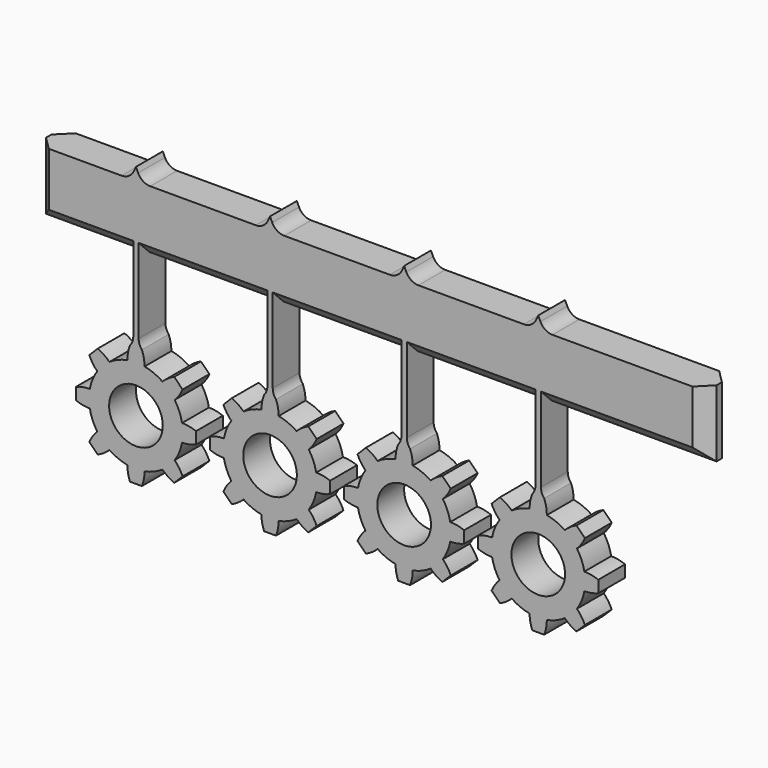
from build123d import *

# Parameters (mm, degrees)
F0_R        = 20
F1_DEPTH    = 12.5
F2_T1_DEPTH = 25
F3_SIZE     = 10


# Not quite as in the source:
# - a fillet or chamfer that OpenCascade refuses, or shapes differently, is made with other operations: its cross-section is extruded or revolved along the edge and cut away or added


with BuildPart() as f1:
    # F0 (on Front) → F1 (new body, symmetric)
    with BuildSketch(Plane.XZ):
        with BuildLine():
            Line((-179.3122274792, 25), (-250, 25))
            Line((-250, 25), (-250, -25))
            Line((-250, -25), (-176.9859883016, -25))
            Line((-176.9859883016, -25), (-176.9859883016, -84.3688530594))
            Line((-176.9859883016, -84.3688530594), (-179.4126922304, -84.3688530594))
            ThreePointArc((-179.4126922304, -84.3688530594), (-180.9081176397, -89.4526936309), (-181.4126922304, -94.727836908))
            ThreePointArc((-181.4126922304, -94.727836908), (-188.3799084344, -96.7969581037), (-194.7695638868, -100.260434299))
            ThreePointArc((-194.7695638868, -100.260434299), (-198.8564415844, -96.8871328307), (-203.5086851747, -94.3497401358))
            Line((-203.5086851747, -94.3497401358), (-209.7689899075, -100.6100448685))
            ThreePointArc((-209.7689899075, -100.6100448685), (-207.2315972126, -105.2622884588), (-203.8582957443, -109.3491661564))
            ThreePointArc((-203.8582957443, -109.3491661564), (-207.3217719395, -115.7388216089), (-209.3908931352, -122.7060378128))
            ThreePointArc((-209.3908931352, -122.7060378128), (-214.6660364123, -123.2106124035), (-219.7498769839, -124.7060378128))
            Line((-219.7498769839, -124.7060378128), (-219.7498769839, -133.5594456704))
            ThreePointArc((-219.7498769839, -133.5594456704), (-214.6660364123, -135.0548710798), (-209.3908931352, -135.5594456704))
            ThreePointArc((-209.3908931352, -135.5594456704), (-207.3217719395, -142.5266618744), (-203.8582957443, -148.9163173268))
            ThreePointArc((-203.8582957443, -148.9163173268), (-207.2315972126, -153.0031950245), (-209.7689899075, -157.6554386148))
            Line((-209.7689899075, -157.6554386148), (-203.5086851747, -163.9157433475))
            ThreePointArc((-203.5086851747, -163.9157433475), (-198.8564415844, -161.3783506526), (-194.7695638868, -158.0050491843))
            ThreePointArc((-194.7695638868, -158.0050491843), (-188.3799084344, -161.4685253795), (-181.4126922304, -163.5376465753))
            ThreePointArc((-181.4126922304, -163.5376465753), (-180.9081176397, -168.8127898524), (-179.4126922304, -173.8966304239))
            Line((-179.4126922304, -173.8966304239), (-170.5592843728, -173.8966304239))
            ThreePointArc((-170.5592843728, -173.8966304239), (-169.0638589634, -168.8127898524), (-168.5592843728, -163.5376465753))
            ThreePointArc((-168.5592843728, -163.5376465753), (-161.5920681688, -161.4685253795), (-155.2024127164, -158.0050491843))
            ThreePointArc((-155.2024127164, -158.0050491843), (-151.1155350188, -161.3783506526), (-146.4632914284, -163.9157433475))
            Line((-146.4632914284, -163.9157433475), (-140.2029866957, -157.6554386148))
            ThreePointArc((-140.2029866957, -157.6554386148), (-142.7403793906, -153.0031950245), (-146.1136808589, -148.9163173268))
            ThreePointArc((-146.1136808589, -148.9163173268), (-142.6502046637, -142.5266618744), (-140.581083468, -135.5594456704))
            ThreePointArc((-140.581083468, -135.5594456704), (-135.3059401909, -135.0548710798), (-130.2220996193, -133.5594456704))
            Line((-130.2220996193, -133.5594456704), (-130.2220996193, -124.7060378128))
            ThreePointArc((-130.2220996193, -124.7060378128), (-135.3059401909, -123.2106124035), (-140.581083468, -122.7060378128))
            ThreePointArc((-140.581083468, -122.7060378128), (-142.6502046637, -115.7388216089), (-146.1136808589, -109.3491661564))
            ThreePointArc((-146.1136808589, -109.3491661564), (-142.7403793906, -105.2622884588), (-140.2029866957, -100.6100448685))
            Line((-140.2029866957, -100.6100448685), (-146.4632914284, -94.3497401358))
            ThreePointArc((-146.4632914284, -94.3497401358), (-151.1155350188, -96.8871328307), (-155.2024127164, -100.260434299))
            ThreePointArc((-155.2024127164, -100.260434299), (-161.5920681688, -96.7969581037), (-168.5592843728, -94.727836908))
            ThreePointArc((-168.5592843728, -94.727836908), (-169.0638589634, -89.4526936309), (-170.5592843728, -84.3688530594))
            Line((-170.5592843728, -84.3688530594), (-172.9859883016, -84.3688530594))
            Line((-172.9859883016, -84.3688530594), (-172.9859883016, -25))
            Line((-172.9859883016, -25), (-76.9859883016, -25))
            Line((-76.9859883016, -25), (-72.9859883016, -25))
            Line((-72.9859883016, -25), (23.0140116984, -25))
            Line((23.0140116984, -25), (23.0140116984, -84.3688530594))
            Line((23.0140116984, -84.3688530594), (20.5873077696, -84.3688530594))
            ThreePointArc((20.5873077696, -84.3688530594), (19.0918823603, -89.4526936309), (18.5873077696, -94.727836908))
            ThreePointArc((18.5873077696, -94.727836908), (11.6200915656, -96.7969581037), (5.2304361132, -100.260434299))
            ThreePointArc((5.2304361132, -100.260434299), (1.1435584156, -96.8871328307), (-3.5086851747, -94.3497401358))
            Line((-3.5086851747, -94.3497401358), (-9.7689899075, -100.6100448685))
            ThreePointArc((-9.7689899075, -100.6100448685), (-7.2315972126, -105.2622884588), (-3.8582957443, -109.3491661564))
            ThreePointArc((-3.8582957443, -109.3491661564), (-7.3217719395, -115.7388216089), (-9.3908931352, -122.7060378128))
            ThreePointArc((-9.3908931352, -122.7060378128), (-14.6660364123, -123.2106124035), (-19.7498769839, -124.7060378128))
            Line((-19.7498769839, -124.7060378128), (-19.7498769839, -133.5594456704))
            ThreePointArc((-19.7498769839, -133.5594456704), (-14.6660364123, -135.0548710798), (-9.3908931352, -135.5594456704))
            ThreePointArc((-9.3908931352, -135.5594456704), (-7.3217719395, -142.5266618744), (-3.8582957443, -148.9163173268))
            ThreePointArc((-3.8582957443, -148.9163173268), (-7.2315972126, -153.0031950245), (-9.7689899075, -157.6554386148))
            Line((-9.7689899075, -157.6554386148), (-3.5086851747, -163.9157433475))
            ThreePointArc((-3.5086851747, -163.9157433475), (1.1435584156, -161.3783506526), (5.2304361132, -158.0050491843))
            ThreePointArc((5.2304361132, -158.0050491843), (11.6200915656, -161.4685253795), (18.5873077696, -163.5376465753))
            ThreePointArc((18.5873077696, -163.5376465753), (19.0918823603, -168.8127898524), (20.5873077696, -173.8966304239))
            Line((20.5873077696, -173.8966304239), (29.4407156272, -173.8966304239))
            ThreePointArc((29.4407156272, -173.8966304239), (30.9361410366, -168.8127898524), (31.4407156272, -163.5376465753))
            ThreePointArc((31.4407156272, -163.5376465753), (38.4079318312, -161.4685253795), (44.7975872836, -158.0050491843))
            ThreePointArc((44.7975872836, -158.0050491843), (48.8844649812, -161.3783506526), (53.5367085716, -163.9157433475))
            Line((53.5367085716, -163.9157433475), (59.7970133043, -157.6554386148))
            ThreePointArc((59.7970133043, -157.6554386148), (57.2596206094, -153.0031950245), (53.8863191411, -148.9163173268))
            ThreePointArc((53.8863191411, -148.9163173268), (57.3497953363, -142.5266618744), (59.418916532, -135.5594456704))
            ThreePointArc((59.418916532, -135.5594456704), (64.6940598091, -135.0548710798), (69.7779003807, -133.5594456704))
            Line((69.7779003807, -133.5594456704), (69.7779003807, -124.7060378128))
            ThreePointArc((69.7779003807, -124.7060378128), (64.6940598091, -123.2106124035), (59.418916532, -122.7060378128))
            ThreePointArc((59.418916532, -122.7060378128), (57.3497953363, -115.7388216089), (53.8863191411, -109.3491661564))
            ThreePointArc((53.8863191411, -109.3491661564), (57.2596206094, -105.2622884588), (59.7970133043, -100.6100448685))
            Line((59.7970133043, -100.6100448685), (53.5367085716, -94.3497401358))
            ThreePointArc((53.5367085716, -94.3497401358), (48.8844649812, -96.8871328307), (44.7975872836, -100.260434299))
            ThreePointArc((44.7975872836, -100.260434299), (38.4079318312, -96.7969581037), (31.4407156272, -94.727836908))
            ThreePointArc((31.4407156272, -94.727836908), (30.9361410366, -89.4526936309), (29.4407156272, -84.3688530594))
            Line((29.4407156272, -84.3688530594), (27.0140116984, -84.3688530594))
            Line((27.0140116984, -84.3688530594), (27.0140116984, -25))
            Line((27.0140116984, -25), (123.0140116984, -25))
            Line((123.0140116984, -25), (123.0140116984, -84.3688530594))
            Line((123.0140116984, -84.3688530594), (120.5873077696, -84.3688530594))
            ThreePointArc((120.5873077696, -84.3688530594), (119.0918823603, -89.4526936309), (118.5873077696, -94.727836908))
            ThreePointArc((118.5873077696, -94.727836908), (111.6200915656, -96.7969581037), (105.2304361132, -100.260434299))
            ThreePointArc((105.2304361132, -100.260434299), (101.1435584156, -96.8871328307), (96.4913148253, -94.3497401358))
            Line((96.4913148253, -94.3497401358), (90.2310100925, -100.6100448685))
            ThreePointArc((90.2310100925, -100.6100448685), (92.7684027874, -105.2622884588), (96.1417042557, -109.3491661564))
            ThreePointArc((96.1417042557, -109.3491661564), (92.6782280605, -115.7388216089), (90.6091068648, -122.7060378128))
            ThreePointArc((90.6091068648, -122.7060378128), (85.3339635877, -123.2106124035), (80.2501230161, -124.7060378128))
            Line((80.2501230161, -124.7060378128), (80.2501230161, -133.5594456704))
            ThreePointArc((80.2501230161, -133.5594456704), (85.3339635877, -135.0548710798), (90.6091068648, -135.5594456704))
            ThreePointArc((90.6091068648, -135.5594456704), (92.6782280605, -142.5266618744), (96.1417042557, -148.9163173268))
            ThreePointArc((96.1417042557, -148.9163173268), (92.7684027874, -153.0031950245), (90.2310100925, -157.6554386148))
            Line((90.2310100925, -157.6554386148), (96.4913148253, -163.9157433475))
            ThreePointArc((96.4913148253, -163.9157433475), (101.1435584156, -161.3783506526), (105.2304361132, -158.0050491843))
            ThreePointArc((105.2304361132, -158.0050491843), (111.6200915656, -161.4685253795), (118.5873077696, -163.5376465753))
            ThreePointArc((118.5873077696, -163.5376465753), (119.0918823603, -168.8127898524), (120.5873077696, -173.8966304239))
            Line((120.5873077696, -173.8966304239), (129.4407156272, -173.8966304239))
            ThreePointArc((129.4407156272, -173.8966304239), (130.9361410366, -168.8127898524), (131.4407156272, -163.5376465753))
            ThreePointArc((131.4407156272, -163.5376465753), (138.4079318312, -161.4685253795), (144.7975872836, -158.0050491843))
            ThreePointArc((144.7975872836, -158.0050491843), (148.8844649812, -161.3783506526), (153.5367085716, -163.9157433475))
            Line((153.5367085716, -163.9157433475), (159.7970133043, -157.6554386148))
            ThreePointArc((159.7970133043, -157.6554386148), (157.2596206094, -153.0031950245), (153.8863191411, -148.9163173268))
            ThreePointArc((153.8863191411, -148.9163173268), (157.3497953363, -142.5266618744), (159.418916532, -135.5594456704))
            ThreePointArc((159.418916532, -135.5594456704), (164.6940598091, -135.0548710798), (169.7779003807, -133.5594456704))
            Line((169.7779003807, -133.5594456704), (169.7779003807, -124.7060378128))
            ThreePointArc((169.7779003807, -124.7060378128), (164.6940598091, -123.2106124035), (159.418916532, -122.7060378128))
            ThreePointArc((159.418916532, -122.7060378128), (157.3497953363, -115.7388216089), (153.8863191411, -109.3491661564))
            ThreePointArc((153.8863191411, -109.3491661564), (157.2596206094, -105.2622884588), (159.7970133043, -100.6100448685))
            Line((159.7970133043, -100.6100448685), (153.5367085716, -94.3497401358))
            ThreePointArc((153.5367085716, -94.3497401358), (148.8844649812, -96.8871328307), (144.7975872836, -100.260434299))
            ThreePointArc((144.7975872836, -100.260434299), (138.4079318312, -96.7969581037), (131.4407156272, -94.727836908))
            ThreePointArc((131.4407156272, -94.727836908), (130.9361410366, -89.4526936309), (129.4407156272, -84.3688530594))
            Line((129.4407156272, -84.3688530594), (127.0140116984, -84.3688530594))
            Line((127.0140116984, -84.3688530594), (127.0140116984, -25))
            Line((127.0140116984, -25), (250, -25))
            Line((250, -25), (250, 25))
            Line((250, 25), (129.340250876, 25))
            Line((129.340250876, 25), (125.0140116984, 34.2776498562))
            Line((125.0140116984, 34.2776498562), (120.6877725208, 25))
            Line((120.6877725208, 25), (29.340250876, 25))
            Line((29.340250876, 25), (25.0140116984, 34.2776498562))
            Line((25.0140116984, 34.2776498562), (20.6877725208, 25))
            Line((20.6877725208, 25), (-70.659749124, 25))
            Line((-70.659749124, 25), (-74.9859883016, 34.2776498562))
            Line((-74.9859883016, 34.2776498562), (-79.3122274792, 25))
            Line((-79.3122274792, 25), (-170.659749124, 25))
            Line((-170.659749124, 25), (-174.9859883016, 34.2776498562))
            Line((-174.9859883016, 34.2776498562), (-179.3122274792, 25))
        make_face()
        with Locations((-174.9859883016, -129.1327417416)):
            Circle(F0_R, mode=Mode.SUBTRACT)
        with Locations((25.0140116984, -129.1327417416)):
            Circle(F0_R, mode=Mode.SUBTRACT)
        with Locations((125.0140116984, -129.1327417416)):
            Circle(F0_R, mode=Mode.SUBTRACT)
        with BuildLine():
            Line((-72.9859883016, -25), (-76.9859883016, -25))
            Line((-76.9859883016, -25), (-76.9859883016, -84.3688530594))
            Line((-76.9859883016, -84.3688530594), (-79.4126922304, -84.3688530594))
            ThreePointArc((-79.4126922304, -84.3688530594), (-80.9081176397, -89.4526936309), (-81.4126922304, -94.727836908))
            ThreePointArc((-81.4126922304, -94.727836908), (-88.3799084344, -96.7969581037), (-94.7695638868, -100.260434299))
            ThreePointArc((-94.7695638868, -100.260434299), (-98.8564415844, -96.8871328307), (-103.5086851747, -94.3497401358))
            Line((-103.5086851747, -94.3497401358), (-109.7689899075, -100.6100448685))
            ThreePointArc((-109.7689899075, -100.6100448685), (-107.2315972126, -105.2622884588), (-103.8582957443, -109.3491661564))
            ThreePointArc((-103.8582957443, -109.3491661564), (-107.3217719395, -115.7388216089), (-109.3908931352, -122.7060378128))
            ThreePointArc((-109.3908931352, -122.7060378128), (-114.6660364123, -123.2106124035), (-119.7498769839, -124.7060378128))
            Line((-119.7498769839, -124.7060378128), (-119.7498769839, -133.5594456704))
            ThreePointArc((-119.7498769839, -133.5594456704), (-114.6660364123, -135.0548710798), (-109.3908931352, -135.5594456704))
            ThreePointArc((-109.3908931352, -135.5594456704), (-107.3217719395, -142.5266618744), (-103.8582957443, -148.9163173268))
            ThreePointArc((-103.8582957443, -148.9163173268), (-107.2315972126, -153.0031950245), (-109.7689899075, -157.6554386148))
            Line((-109.7689899075, -157.6554386148), (-103.5086851747, -163.9157433475))
            ThreePointArc((-103.5086851747, -163.9157433475), (-98.8564415844, -161.3783506526), (-94.7695638868, -158.0050491843))
            ThreePointArc((-94.7695638868, -158.0050491843), (-88.3799084344, -161.4685253795), (-81.4126922304, -163.5376465753))
            ThreePointArc((-81.4126922304, -163.5376465753), (-80.9081176397, -168.8127898524), (-79.4126922304, -173.8966304239))
            Line((-79.4126922304, -173.8966304239), (-70.5592843728, -173.8966304239))
            ThreePointArc((-70.5592843728, -173.8966304239), (-69.0638589634, -168.8127898524), (-68.5592843728, -163.5376465753))
            ThreePointArc((-68.5592843728, -163.5376465753), (-61.5920681688, -161.4685253795), (-55.2024127164, -158.0050491843))
            ThreePointArc((-55.2024127164, -158.0050491843), (-51.1155350188, -161.3783506526), (-46.4632914284, -163.9157433475))
            Line((-46.4632914284, -163.9157433475), (-40.2029866957, -157.6554386148))
            ThreePointArc((-40.2029866957, -157.6554386148), (-42.7403793906, -153.0031950245), (-46.1136808589, -148.9163173268))
            ThreePointArc((-46.1136808589, -148.9163173268), (-42.6502046637, -142.5266618744), (-40.581083468, -135.5594456704))
            ThreePointArc((-40.581083468, -135.5594456704), (-35.3059401909, -135.0548710798), (-30.2220996193, -133.5594456704))
            Line((-30.2220996193, -133.5594456704), (-30.2220996193, -124.7060378128))
            ThreePointArc((-30.2220996193, -124.7060378128), (-35.3059401909, -123.2106124035), (-40.581083468, -122.7060378128))
            ThreePointArc((-40.581083468, -122.7060378128), (-42.6502046637, -115.7388216089), (-46.1136808589, -109.3491661564))
            ThreePointArc((-46.1136808589, -109.3491661564), (-42.7403793906, -105.2622884588), (-40.2029866957, -100.6100448685))
            Line((-40.2029866957, -100.6100448685), (-46.4632914284, -94.3497401358))
            ThreePointArc((-46.4632914284, -94.3497401358), (-51.1155350188, -96.8871328307), (-55.2024127164, -100.260434299))
            ThreePointArc((-55.2024127164, -100.260434299), (-61.5920681688, -96.7969581037), (-68.5592843728, -94.727836908))
            ThreePointArc((-68.5592843728, -94.727836908), (-69.0638589634, -89.4526936309), (-70.5592843728, -84.3688530594))
            Line((-70.5592843728, -84.3688530594), (-72.9859883016, -84.3688530594))
            Line((-72.9859883016, -84.3688530594), (-72.9859883016, -25))
        make_face()
        with Locations((-74.9859883016, -129.1327417416)):
            Circle(F0_R, mode=Mode.SUBTRACT)
    extrude(amount=F1_DEPTH, both=True)

    # F2: fillet of radius 10 on 16 edges, made by hand

    # F2_s2 → F2_t1 (join)
    with BuildSketch(Plane.XZ.offset(-12.5)):
        with BuildLine():
            ThreePointArc((-185.6829300873, 25), (-180.3099340038, 26.5660855419), (-176.6198522169, 30.7738173826))
            Line((-176.6198522169, 30.7738173826), (-179.3122274792, 25))
            Line((-179.3122274792, 25), (-185.6829300873, 25))
        make_face()
        with BuildLine():
            ThreePointArc((-179.4126922304, -84.3688530594), (-177.6122761044, -81.3218450467), (-176.9859883016, -77.8385248427))
            Line((-176.9859883016, -77.8385248427), (-176.9859883016, -84.3688530594))
            Line((-176.9859883016, -84.3688530594), (-179.4126922304, -84.3688530594))
        make_face()
        with BuildLine():
            ThreePointArc((-85.6829300873, 25), (-80.3099340038, 26.5660855419), (-76.6198522169, 30.7738173826))
            Line((-76.6198522169, 30.7738173826), (-79.3122274792, 25))
            Line((-79.3122274792, 25), (-85.6829300873, 25))
        make_face()
        with BuildLine():
            ThreePointArc((14.3170699127, 25), (19.6900659962, 26.5660855419), (23.3801477831, 30.7738173826))
            Line((23.3801477831, 30.7738173826), (20.6877725208, 25))
            Line((20.6877725208, 25), (14.3170699127, 25))
        make_face()
        with BuildLine():
            ThreePointArc((114.3170699127, 25), (119.6900659962, 26.5660855419), (123.3801477831, 30.7738173826))
            Line((123.3801477831, 30.7738173826), (120.6877725208, 25))
            Line((120.6877725208, 25), (114.3170699127, 25))
        make_face()
        with BuildLine():
            ThreePointArc((120.5873077696, -84.3688530594), (122.3877238956, -81.3218450467), (123.0140116984, -77.8385248427))
            Line((123.0140116984, -77.8385248427), (123.0140116984, -84.3688530594))
            Line((123.0140116984, -84.3688530594), (120.5873077696, -84.3688530594))
        make_face()
        with BuildLine():
            ThreePointArc((20.5873077696, -84.3688530594), (22.3877238956, -81.3218450467), (23.0140116984, -77.8385248427))
            Line((23.0140116984, -77.8385248427), (23.0140116984, -84.3688530594))
            Line((23.0140116984, -84.3688530594), (20.5873077696, -84.3688530594))
        make_face()
        with BuildLine():
            ThreePointArc((-79.4126922304, -84.3688530594), (-77.6122761044, -81.3218450467), (-76.9859883016, -77.8385248427))
            Line((-76.9859883016, -77.8385248427), (-76.9859883016, -84.3688530594))
            Line((-76.9859883016, -84.3688530594), (-79.4126922304, -84.3688530594))
        make_face()
        with BuildLine():
            ThreePointArc((-173.3521243862, 30.7738173826), (-169.6620425993, 26.5660855419), (-164.2890465159, 25))
            Line((-164.2890465159, 25), (-170.659749124, 25))
            Line((-170.659749124, 25), (-173.3521243862, 30.7738173826))
        make_face()
        with BuildLine():
            ThreePointArc((-73.3521243862, 30.7738173826), (-69.6620425993, 26.5660855419), (-64.2890465159, 25))
            Line((-64.2890465159, 25), (-70.659749124, 25))
            Line((-70.659749124, 25), (-73.3521243862, 30.7738173826))
        make_face()
        with BuildLine():
            ThreePointArc((26.6478756138, 30.7738173826), (30.3379574007, 26.5660855419), (35.7109534841, 25))
            Line((35.7109534841, 25), (29.340250876, 25))
            Line((29.340250876, 25), (26.6478756138, 30.7738173826))
        make_face()
        with BuildLine():
            ThreePointArc((126.6478756138, 30.7738173826), (130.3379574007, 26.5660855419), (135.7109534841, 25))
            Line((135.7109534841, 25), (129.340250876, 25))
            Line((129.340250876, 25), (126.6478756138, 30.7738173826))
        make_face()
        with BuildLine():
            ThreePointArc((-72.9859883016, -77.8385248427), (-72.3597004988, -81.3218450467), (-70.5592843728, -84.3688530594))
            Line((-70.5592843728, -84.3688530594), (-72.9859883016, -84.3688530594))
            Line((-72.9859883016, -84.3688530594), (-72.9859883016, -77.8385248427))
        make_face()
        with BuildLine():
            ThreePointArc((-172.9859883016, -77.8385248427), (-172.3597004988, -81.3218450467), (-170.5592843728, -84.3688530594))
            Line((-170.5592843728, -84.3688530594), (-172.9859883016, -84.3688530594))
            Line((-172.9859883016, -84.3688530594), (-172.9859883016, -77.8385248427))
        make_face()
        with BuildLine():
            ThreePointArc((27.0140116984, -77.8385248427), (27.6402995012, -81.3218450467), (29.4407156272, -84.3688530594))
            Line((29.4407156272, -84.3688530594), (27.0140116984, -84.3688530594))
            Line((27.0140116984, -84.3688530594), (27.0140116984, -77.8385248427))
        make_face()
        with BuildLine():
            ThreePointArc((129.4407156272, -84.3688530594), (127.6402995012, -81.3218450467), (127.0140116984, -77.8385248427))
            Line((127.0140116984, -77.8385248427), (127.0140116984, -84.3688530594))
            Line((127.0140116984, -84.3688530594), (129.4407156272, -84.3688530594))
        make_face()
    extrude(amount=F2_T1_DEPTH)

    # F3
    f3_edges = [f1.edges().sort_by_distance(p)[0] for p in [
        (-250, -12.5, 0),
        (-213.492994, -12.5, -25),
        (-124.985988, -12.5, -25),
        (-24.985988, -12.5, -25),
        (75.014012, -12.5, -25),
        (188.507006, -12.5, -25),
        (250, 12.5, 0),
        (-250, 12.5, 0),
        (-213.492994, 12.5, -25),
        (-124.985988, 12.5, -25),
        (188.507006, 12.5, -25),
        (75.014012, 12.5, -25),
        (-24.985988, 12.5, -25),
        (250, -12.5, 0),
    ]]
    chamfer(f3_edges, length=F3_SIZE)


solid = f1.part
